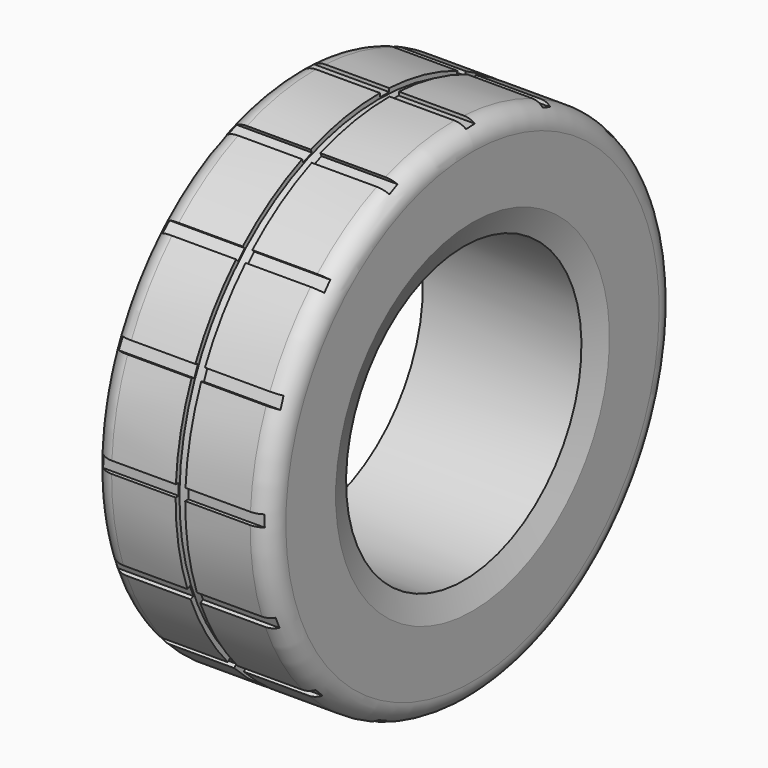
from build123d import *

# Parameters (mm, degrees)
F3_W     = 224.2247087342
F3_H     = 12
F4_DEPTH = 25
F8_COUNT = 16


# Not quite as in the source:
# - a feature of the source that left no trace in its solid (it failed there, or was rolled back) is left out


with BuildPart() as f1:
    # F0 (on Front) → F1 (revolve)
    with BuildSketch(Plane.XZ):
        with BuildLine():
            Line((-92.5, 178), (-82.5, 153))
            Line((-82.5, 153), (82.5, 153))
            Line((82.5, 153), (91.5637493134, 178))
            Line((91.5637493134, 178), (91.5637493134, 242.6291943789))
            ThreePointArc((91.5637493134, 242.6291943789), (86.2295393168, 257.648880679), (71.6107823172, 264))
            Line((71.6107823172, 264), (4.0637493134, 264))
            Line((4.0637493134, 264), (4.0637493134, 259))
            Line((4.0637493134, 259), (-5.9362506866, 259))
            Line((-5.9362506866, 259), (-5.9362506866, 264))
            Line((-5.9362506866, 264), (-72.5, 264))
            ThreePointArc((-72.5, 264), (-86.6421356237, 258.1421356237), (-92.5, 244))
            Line((-92.5, 244), (-92.5, 178))
        make_face()
    revolve(axis=Axis((-3.5022934647, 0, 0), (1, 0, 0)))

    # F3 (on offset) → F4 (cut)
    with BuildSketch(Plane.XY.offset(260)):
        with Locations((0.8777305484, 7.5715146959)):
            Rectangle(F3_W, F3_H)
    f4 = extrude(amount=F4_DEPTH, mode=Mode.SUBTRACT)


with BuildPart() as f5_1:
    # F5: copy of F1
    add(f1.part)


with BuildPart() as f1_1:
    add(f1.part)

    # F8: F4 ×16 about axis
    f8_axis = Axis((-92.5, 0, 0), (1, 0, 0))
    for i in range(1, F8_COUNT):
        add(f4.rotate(f8_axis, i * 360 / F8_COUNT), mode=Mode.SUBTRACT)


solid = f1_1.part
